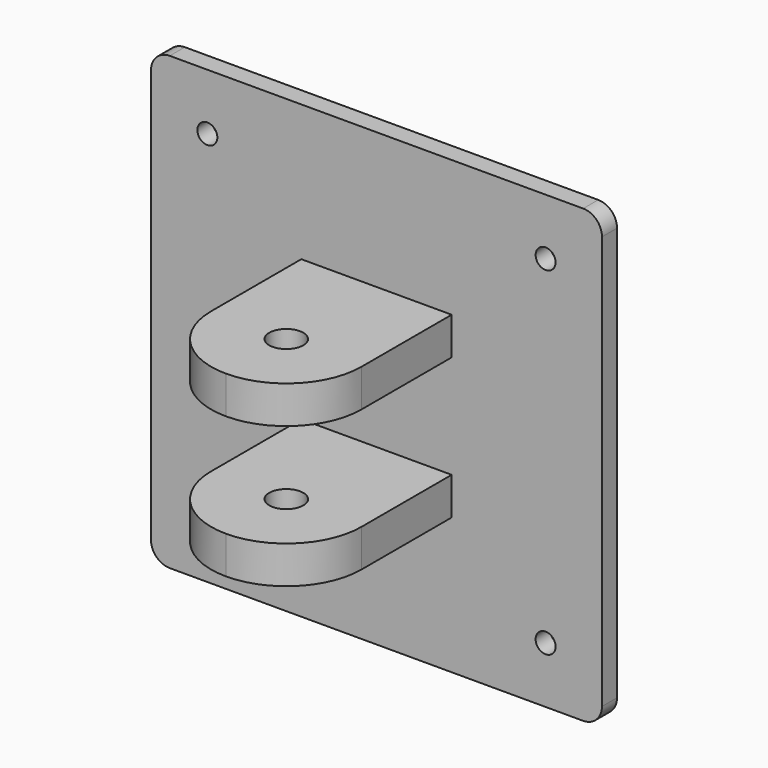
from build123d import *

# Parameters (mm, degrees)
F0_W     = 152.4
F0_H     = 152.4
F1_DEPTH = 6.35
F2_W     = 50.8
F2_H     = 12.7
F3_DEPTH = 63.5
F4_R     = 5.7546875
F5_DEPTH = 76.2
F6_R     = 3.3734375
F7_DEPTH = 6.35
F8_R     = 25.39999
F8_2_R   = 25.39999
F9_R     = 6.35


# Not quite as in the source:
# - a fillet or chamfer is up to 0.001 mm smaller than in the source, because OpenCascade refuses the exact size


with BuildPart() as f1:
    # F0 (on Front) → F1 (new body)
    with BuildSketch(Plane.XZ):
        with Locations((76.2, 76.2)):
            Rectangle(F0_W, F0_H)
    extrude(amount=F1_DEPTH)

    # F6 (on face) → F7 (cut)
    with BuildSketch(Plane.XZ.offset(6.35)):
        with Locations((19.05, 133.35)):
            Circle(F6_R)
        with Locations((133.35, 133.35)):
            Circle(F6_R)
        with Locations((19.05, 19.05)):
            Circle(F6_R)
        with Locations((133.35, 19.05)):
            Circle(F6_R)
    extrude(amount=-F7_DEPTH, mode=Mode.SUBTRACT)

    # F9
    f9_edges = [f1.edges().sort_by_distance(p)[0] for p in [
        (0, -3.175, 152.4),
        (152.4, -3.175, 152.4),
        (0, -3.175, 0),
        (152.4, -3.175, 0),
    ]]
    fillet(f9_edges, radius=F9_R)


with BuildPart() as f3:
    # F2 (on face) → F3 (new body)
    with BuildSketch(Plane.XZ.offset(6.35)):
        with Locations((76.2, 100.0125)):
            Rectangle(F2_W, F2_H)
    extrude(amount=F3_DEPTH)


with BuildPart() as f3b:
    # F2 (on face) → F3, piece 2 (new body)
    with BuildSketch(Plane.XZ.offset(6.35)):
        with Locations((76.2, 52.3875)):
            Rectangle(F2_W, F2_H)
    extrude(amount=F3_DEPTH)


with BuildPart() as f5_tool:
    # F4 (on face) → F5 (new body)
    with BuildSketch(Plane.XY.offset(106.3625)):
        with Locations((76.2, -44.45)):
            Circle(F4_R)
    extrude(amount=-F5_DEPTH)


with BuildPart() as f3_1:
    add(f3.part)

    # F5: cut by f5_tool
    add(f5_tool.part, mode=Mode.SUBTRACT)

    # F8 (radius 25.4 in the source; OpenCascade refuses exactly that, so slightly less here)
    f8_edges = [f3_1.edges().sort_by_distance(p)[0] for p in [
        (50.8, -69.85, 100.0125),
        (101.6, -69.85, 100.0125),
    ]]
    fillet(f8_edges, radius=F8_R)


with BuildPart() as f3b_1:
    add(f3b.part)

    # F5: cut by f5_tool
    add(f5_tool.part, mode=Mode.SUBTRACT)

    # F8#2 (radius 25.4 in the source; OpenCascade refuses exactly that, so slightly less here)
    f8_2_edges = [f3b_1.edges().sort_by_distance(p)[0] for p in [
        (50.8, -69.85, 52.3875),
        (101.6, -69.85, 52.3875),
    ]]
    fillet(f8_2_edges, radius=F8_2_R)


solid = Compound([f1.part, f3_1.part, f3b_1.part])
